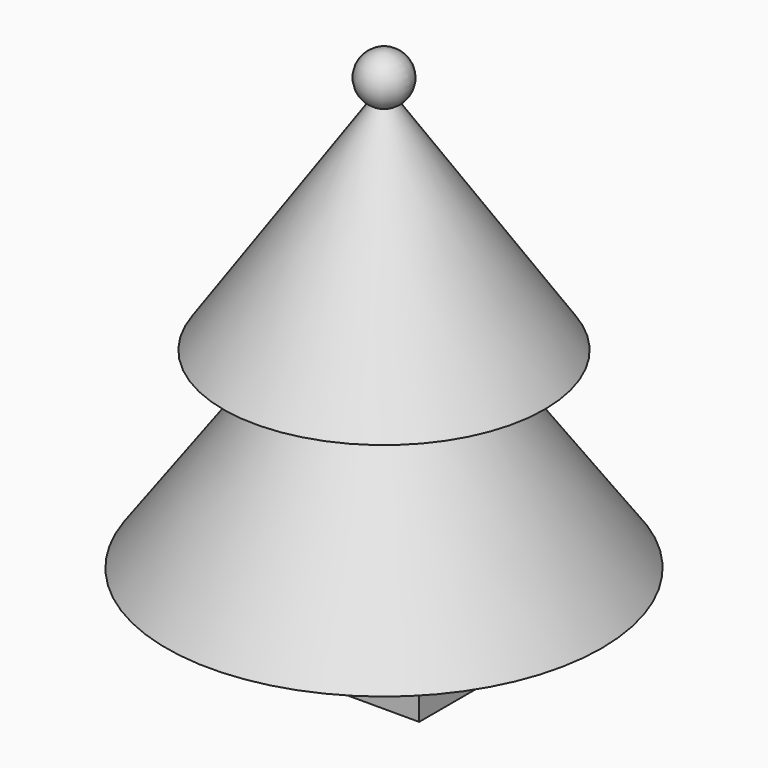
from build123d import *

# Parameters (mm, degrees)
F0_W     = 4.3170871213
F0_H     = 8.0585610121
F2_W     = 21.2777061388
F2_H     = 17.4885243177
F3_DEPTH = 2.54


# Not quite as in the source:
# - a feature names something its author has since deleted; it is built from what else it names


with BuildPart() as f1:
    # F0 (on Front) → F1 (revolve)
    with BuildSketch(Plane.XZ):
        Polygon((8.9219789952, 29.3561872095), (0, 29.3561872095), (0, 8.0585610121), (4.3170871213, 8.0585610121), (24.1756830364, 8.0585610121), align=None)
        with Locations((2.1585435607, 4.0292805061)):
            Rectangle(F0_W, F0_H)
        with BuildLine():
            Line((17.8439579904, 29.3561872095), (1.3134449127, 53.6187163612))
            ThreePointArc((1.3134449127, 53.6187163612), (0.6772695352, 53.3730420313), (0, 53.2931610942))
            Line((0, 53.2931610942), (0, 29.3561872095))
            Line((0, 29.3561872095), (8.9219789952, 29.3561872095))
            Line((8.9219789952, 29.3561872095), (17.8439579904, 29.3561872095))
        make_face()
    revolve(axis=Axis((0, 0, 0.1439042389), (0, 0, -1)))

    # F2 (on Top) → F3 (join)
    with BuildSketch(Plane.XY):
        with Locations((0.1457375474, 0.1457380131)):
            Rectangle(F2_W, F2_H)
    extrude(amount=F3_DEPTH)


with BuildPart() as f1b:
    # F0 (on Front) → F1, piece 2 (revolve)
    with BuildSketch(Plane.XZ):
        with BuildLine():
            Line((0, 58.7384924293), (0, 55.5465146899))
            Line((0, 55.5465146899), (1.3134449127, 53.6187163612))
            ThreePointArc((1.3134449127, 53.6187163612), (2.6595703819, 56.6924218716), (0, 58.7384924293))
        make_face()
    revolve(axis=Axis((0, 0, 0.1439042389), (0, 0, -1)))


solid = Compound([f1.part, f1b.part])
